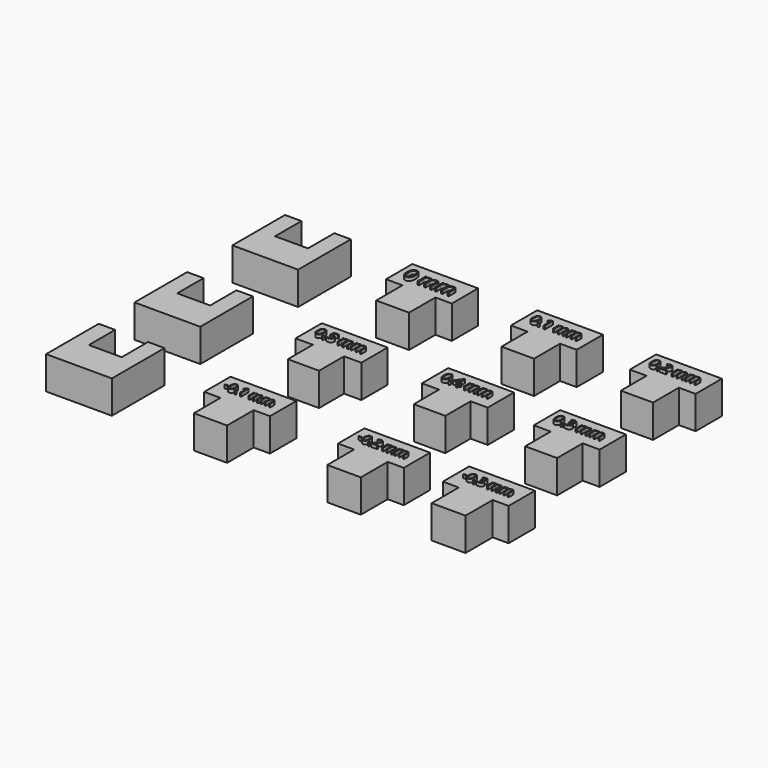
from build123d import *

# Parameters (mm, degrees)
F1_DEPTH      = 10
F2_TEXT_SIZE  = 5.6061667835
F3_DEPTH      = 1
F4_TEXT_SIZE  = 4.2693231344
F5_DEPTH      = 1
F6_TEXT_SIZE  = 4.2693231344
F7_DEPTH      = 1
F8_TEXT_SIZE  = 4.2693231344
F9_DEPTH      = 1
F10_TEXT_SIZE = 4.2693231344
F11_DEPTH     = 1
F12_TEXT_SIZE = 4.2693231344
F13_DEPTH     = 1
F14_TEXT_SIZE = 3.9111835404
F15_DEPTH     = 1
F16_TEXT_SIZE = 3.9111835404
F17_DEPTH     = 1
F18_TEXT_SIZE = 3.9111835404
F19_DEPTH     = 1


# Not quite as in the source:
# - Text() gives the source's letters only with a copy of the font that has no kerning and outlines rounded to 1/6400 em; it was checked with that copy


with BuildPart() as f1:
    # F0 (on Top) → F1 (new body)
    with BuildSketch(Plane.XY):
        Polygon((-56.9452023506, 43.8183426622), (-61.9452023506, 43.8183426622), (-61.9452023506, 23.8183426622), (-41.9452023506, 23.8183426622), (-41.9452023506, 43.8183426622), (-46.9452023506, 43.8183426622), (-46.9452023506, 33.8183426622), (-56.9452023506, 33.8183426622), align=None)
    extrude(amount=F1_DEPTH)


with BuildPart() as f1b:
    # F0 (on Top) → F1, piece 2 (new body)
    with BuildSketch(Plane.XY):
        Polygon((-22.5773579441, 33.0135617405), (-17.5773579441, 33.0135617405), (-17.5773579441, 23.0135617405), (-7.5773579441, 23.0135617405), (-7.5773579441, 33.0135617405), (-2.5773579441, 33.0135617405), (-2.5773579441, 43.0135617405), (-22.5773579441, 43.0135617405), align=None)
    extrude(amount=F1_DEPTH)

    # F2 (on face) → F3 (join)
    with BuildSketch(Plane.XY.offset(10)):
        with Locations((-20.0773579441, 35.4771216564)):
            Text('0 mm', F2_TEXT_SIZE, font='Open Sans', text_align=(TextAlign.LEFT, TextAlign.BOTTOM))
    extrude(amount=F3_DEPTH)


with BuildPart() as f1c:
    # F0 (on Top) → F1, piece 3 (new body)
    with BuildSketch(Plane.XY):
        Polygon((15.4259026838, 32.9628368528), (20.4759026838, 32.9628368528), (20.4759026838, 23.0628368528), (30.3759026838, 23.0628368528), (30.3759026838, 32.9628368528), (35.4259026838, 32.9628368528), (35.4259026838, 42.9628368528), (15.4259026838, 42.9628368528), align=None)
    extrude(amount=F1_DEPTH)

    # F4 (on face) → F5 (join)
    with BuildSketch(Plane.XY.offset(10)):
        with Locations((17.9259026838, 36.388924196)):
            Text('0.1 mm', F4_TEXT_SIZE, font='Open Sans', text_align=(TextAlign.LEFT, TextAlign.BOTTOM))
    extrude(amount=F5_DEPTH)


with BuildPart() as f1d:
    # F0 (on Top) → F1, piece 4 (new body)
    with BuildSketch(Plane.XY):
        Polygon((51.633169651, 32.8925785896), (56.733169651, 32.8925785896), (56.733169651, 23.0925785896), (66.533169651, 23.0925785896), (66.533169651, 32.8925785896), (71.633169651, 32.8925785896), (71.633169651, 42.8925785896), (51.633169651, 42.8925785896), align=None)
    extrude(amount=F1_DEPTH)

    # F6 (on face) → F7 (join)
    with BuildSketch(Plane.XY.offset(10)):
        with Locations((54.133169651, 36.3186659329)):
            Text('0.2 mm', F6_TEXT_SIZE, font='Open Sans', text_align=(TextAlign.LEFT, TextAlign.BOTTOM))
    extrude(amount=F7_DEPTH)


with BuildPart() as f1e:
    # F0 (on Top) → F1, piece 5 (new body)
    with BuildSketch(Plane.XY):
        Polygon((51.728592962, -3.7110992652), (56.878592962, -3.7110992652), (56.878592962, -13.4110992652), (66.578592962, -13.4110992652), (66.578592962, -3.7110992652), (71.728592962, -3.7110992652), (71.728592962, 6.2889007348), (51.728592962, 6.2889007348), align=None)
    extrude(amount=F1_DEPTH)

    # F12 (on face) → F13 (join)
    with BuildSketch(Plane.XY.offset(10)):
        with Locations((54.228592962, -0.285011922)):
            Text('0.3 mm', F12_TEXT_SIZE, font='Open Sans', text_align=(TextAlign.LEFT, TextAlign.BOTTOM))
    extrude(amount=F13_DEPTH)


with BuildPart() as f1f:
    # F0 (on Top) → F1, piece 6 (new body)
    with BuildSketch(Plane.XY):
        Polygon((17.496650815, -3.4446209112), (22.696650815, -3.4446209112), (22.696650815, -13.0446209112), (32.296650815, -13.0446209112), (32.296650815, -3.4446209112), (37.496650815, -3.4446209112), (37.496650815, 6.5553790888), (17.496650815, 6.5553790888), align=None)
    extrude(amount=F1_DEPTH)

    # F10 (on face) → F11 (join)
    with BuildSketch(Plane.XY.offset(10)):
        with Locations((19.996650815, -0.0185335679)):
            Text('0.4 mm', F10_TEXT_SIZE, font='Open Sans', text_align=(TextAlign.LEFT, TextAlign.BOTTOM))
    extrude(amount=F11_DEPTH)


with BuildPart() as f1g:
    # F0 (on Top) → F1, piece 7 (new body)
    with BuildSketch(Plane.XY):
        Polygon((-20.3525044397, -4.1576060165), (-15.1025044397, -4.1576060165), (-15.1025044397, -13.6576060165), (-5.6025044397, -13.6576060165), (-5.6025044397, -4.1576060165), (-0.3525044397, -4.1576060165), (-0.3525044397, 5.8423939835), (-20.3525044397, 5.8423939835), align=None)
    extrude(amount=F1_DEPTH)

    # F8 (on face) → F9 (join)
    with BuildSketch(Plane.XY.offset(10)):
        with Locations((-17.8525044397, -0.7315186733)):
            Text('0.5 mm', F8_TEXT_SIZE, font='Open Sans', text_align=(TextAlign.LEFT, TextAlign.BOTTOM))
    extrude(amount=F9_DEPTH)


with BuildPart() as f1h:
    # F0 (on Top) → F1, piece 8 (new body)
    with BuildSketch(Plane.XY):
        Polygon((-20.1091777906, -39.1814293651), (-15.1591777906, -39.1814293651), (-15.1591777906, -49.2814293651), (-5.0591777906, -49.2814293651), (-5.0591777906, -39.1814293651), (-0.1091777906, -39.1814293651), (-0.1091777906, -29.1814293651), (-20.1091777906, -29.1814293651), align=None)
    extrude(amount=F1_DEPTH)

    # F14 (on face) → F15 (join)
    with BuildSketch(Plane.XY.offset(10)):
        with Locations((-17.6091777906, -35.6814293651)):
            Text('-0.1 mm', F14_TEXT_SIZE, font='Open Sans', text_align=(TextAlign.LEFT, TextAlign.BOTTOM))
    extrude(amount=F15_DEPTH)


with BuildPart() as f1i:
    # F0 (on Top) → F1, piece 9 (new body)
    with BuildSketch(Plane.XY):
        Polygon((21.2893874943, -40.0706754562), (26.1893874943, -40.0706754562), (26.1893874943, -50.2706754562), (36.3893874943, -50.2706754562), (36.3893874943, -40.0706754562), (41.2893874943, -40.0706754562), (41.2893874943, -30.0706754562), (21.2893874943, -30.0706754562), align=None)
    extrude(amount=F1_DEPTH)

    # F16 (on face) → F17 (join)
    with BuildSketch(Plane.XY.offset(10)):
        with Locations((23.7893874943, -36.5706754562)):
            Text('-0.2 mm', F16_TEXT_SIZE, font='Open Sans', text_align=(TextAlign.LEFT, TextAlign.BOTTOM))
    extrude(amount=F17_DEPTH)


with BuildPart() as f1j:
    # F0 (on Top) → F1, piece 10 (new body)
    with BuildSketch(Plane.XY):
        Polygon((52.945716083, -39.8167642613), (57.795716083, -39.8167642613), (57.795716083, -50.1167642613), (68.095716083, -50.1167642613), (68.095716083, -39.8167642613), (72.945716083, -39.8167642613), (72.945716083, -29.8167642613), (52.945716083, -29.8167642613), align=None)
    extrude(amount=F1_DEPTH)

    # F18 (on face) → F19 (join)
    with BuildSketch(Plane.XY.offset(10)):
        with Locations((55.445716083, -36.3167642613)):
            Text('-0.3 mm', F18_TEXT_SIZE, font='Open Sans', text_align=(TextAlign.LEFT, TextAlign.BOTTOM))
    extrude(amount=F19_DEPTH)


with BuildPart() as f1k:
    # F0 (on Top) → F1, piece 11 (new body)
    with BuildSketch(Plane.XY):
        Polygon((-56.7543080263, 6.3892710485), (-61.7543080263, 6.3892710485), (-61.7543080263, -13.6107289515), (-41.7543080263, -13.6107289515), (-41.7543080263, 6.3892710485), (-46.7543080263, 6.3892710485), (-46.7543080263, -3.6107289515), (-56.7543080263, -3.6107289515), align=None)
    extrude(amount=F1_DEPTH)


with BuildPart() as f1l:
    # F0 (on Top) → F1, piece 12 (new body)
    with BuildSketch(Plane.XY):
        Polygon((-56.5391658398, -27.4763673153), (-61.5391658398, -27.4763673153), (-61.5391658398, -47.4763673153), (-41.5391658398, -47.4763673153), (-41.5391658398, -27.4763673153), (-46.5391658398, -27.4763673153), (-46.5391658398, -37.4763673153), (-56.5391658398, -37.4763673153), align=None)
    extrude(amount=F1_DEPTH)


solid = Compound([f1.part, f1b.part, f1c.part, f1d.part, f1e.part, f1f.part, f1g.part, f1h.part, f1i.part, f1j.part, f1k.part, f1l.part])
